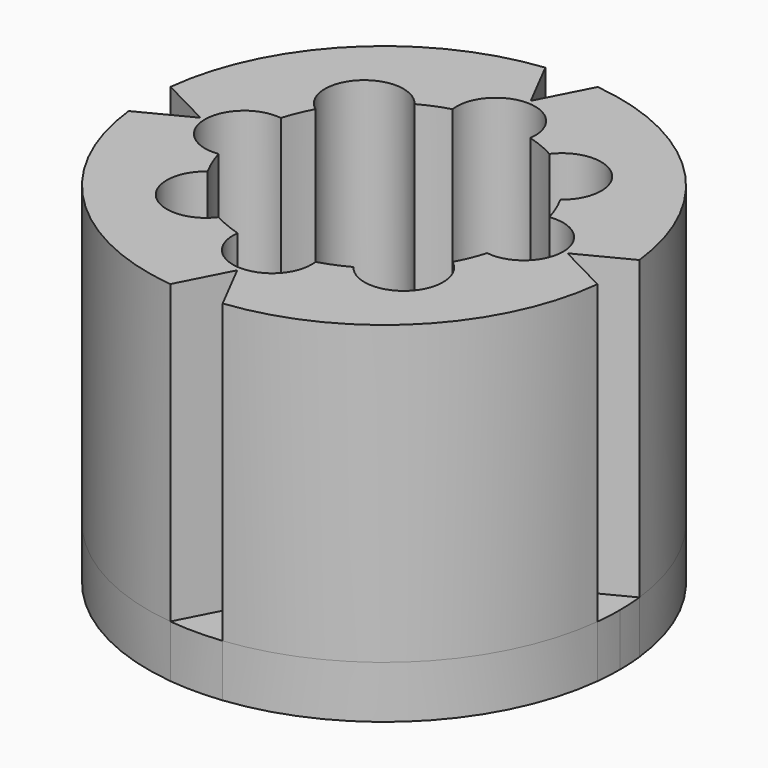
from build123d import *
from build123d import SkipClean  # not in build123d's __all__

# Parameters (mm, degrees)
F0_R     = 1.25
F0_R_2   = 4.5
F1_DEPTH = 20
F3_DEPTH = 19
F4_R     = 13.5
F4_R_2   = 10.5
F5_DEPTH = 3


with BuildPart() as f1:
    # F0 (on Top) → F1 (new body)
    with BuildSketch(Plane.XY):
        with BuildLine():
            Line((-10.5, 0), (-13.416407865, -1.5))
            ThreePointArc((-13.416407865, -1.5), (-9.545941546, -9.545941546), (-1.5, -13.416407865))
            Line((-1.5, -13.416407865), (0, -10.5))
            Line((0, -10.5), (1.5, -13.416407865))
            ThreePointArc((1.5, -13.416407865), (9.545941546, -9.545941546), (13.416407865, -1.5))
            Line((13.416407865, -1.5), (10.5, 0))
            Line((10.5, 0), (13.416407865, 1.5))
            ThreePointArc((13.416407865, 1.5), (9.545941546, 9.545941546), (1.5, 13.416407865))
            Line((1.5, 13.416407865), (0, 10.5))
            Line((0, 10.5), (-1.5, 13.416407865))
            ThreePointArc((-1.5, 13.416407865), (-9.545941546, 9.545941546), (-13.416407865, 1.5))
            Line((-13.416407865, 1.5), (-10.5, 0))
        make_face()
        with Locations((-5.6568542495, -5.6568542495)):
            Circle(F0_R, mode=Mode.SUBTRACT)
        with Locations((0, -8)):
            Circle(F0_R, mode=Mode.SUBTRACT)
        with Locations((5.6568542495, -5.6568542495)):
            Circle(F0_R, mode=Mode.SUBTRACT)
        with Locations((-8, 0)):
            Circle(F0_R, mode=Mode.SUBTRACT)
        with Locations((-5.6568542495, 5.6568542495)):
            Circle(F0_R, mode=Mode.SUBTRACT)
        Circle(F0_R_2, mode=Mode.SUBTRACT)
        with Locations((5.6568542495, 5.6568542495)):
            Circle(F0_R, mode=Mode.SUBTRACT)
        with Locations((8, 0)):
            Circle(F0_R, mode=Mode.SUBTRACT)
        with Locations((0, 8)):
            Circle(F0_R, mode=Mode.SUBTRACT)
    extrude(amount=F1_DEPTH)

    # F2 (on face) → F3 (cut)
    with BuildSketch(Plane.XY.offset(20)):
        with BuildLine():
            ThreePointArc((-7.0083017238, 3.8579407652), (-7.3910362601, 3.0614674589), (-7.68359375, 2.2276415971))
            ThreePointArc((-7.68359375, 2.2276415971), (-10.25, 0), (-7.68359375, -2.2276415971))
            ThreePointArc((-7.68359375, -2.2276415971), (-7.3910362601, -3.0614674589), (-7.0083017238, -3.8579407652))
            ThreePointArc((-7.0083017238, -3.8579407652), (-7.2478445072, -7.2478445072), (-3.8579407652, -7.0083017238))
            ThreePointArc((-3.8579407652, -7.0083017238), (-3.0614674589, -7.3910362601), (-2.2276415971, -7.68359375))
            ThreePointArc((-2.2276415971, -7.68359375), (0, -10.25), (2.2276415971, -7.68359375))
            ThreePointArc((2.2276415971, -7.68359375), (3.0614674589, -7.3910362601), (3.8579407652, -7.0083017238))
            ThreePointArc((3.8579407652, -7.0083017238), (7.2478445072, -7.2478445072), (7.0083017238, -3.8579407652))
            ThreePointArc((7.0083017238, -3.8579407652), (7.3910362601, -3.0614674589), (7.68359375, -2.2276415971))
            ThreePointArc((7.68359375, -2.2276415971), (10.25, 0), (7.68359375, 2.2276415971))
            ThreePointArc((7.68359375, 2.2276415971), (7.3910362601, 3.0614674589), (7.0083017238, 3.8579407652))
            ThreePointArc((7.0083017238, 3.8579407652), (7.2478445072, 7.2478445072), (3.8579407652, 7.0083017238))
            ThreePointArc((3.8579407652, 7.0083017238), (3.0614674589, 7.3910362601), (2.2276415971, 7.68359375))
            ThreePointArc((2.2276415971, 7.68359375), (0, 10.25), (-2.2276415971, 7.68359375))
            ThreePointArc((-2.2276415971, 7.68359375), (-3.0614674589, 7.3910362601), (-3.8579407652, 7.0083017238))
            ThreePointArc((-3.8579407652, 7.0083017238), (-7.2478445072, 7.2478445072), (-7.0083017238, 3.8579407652))
        make_face()
    extrude(amount=-F3_DEPTH, mode=Mode.SUBTRACT)

    # F4 (on face) → F5 (join)
    with BuildSketch(Plane(origin=(0, 0, 0), x_dir=(1, 0, 0), z_dir=(0, 0, -1))):
        Circle(F4_R)
        Circle(F4_R_2, mode=Mode.SUBTRACT)
    with SkipClean():  # cleaning this boolean's faces spoils the solid; the shape is the same uncleaned
        extrude(amount=-F5_DEPTH)


solid = f1.part
